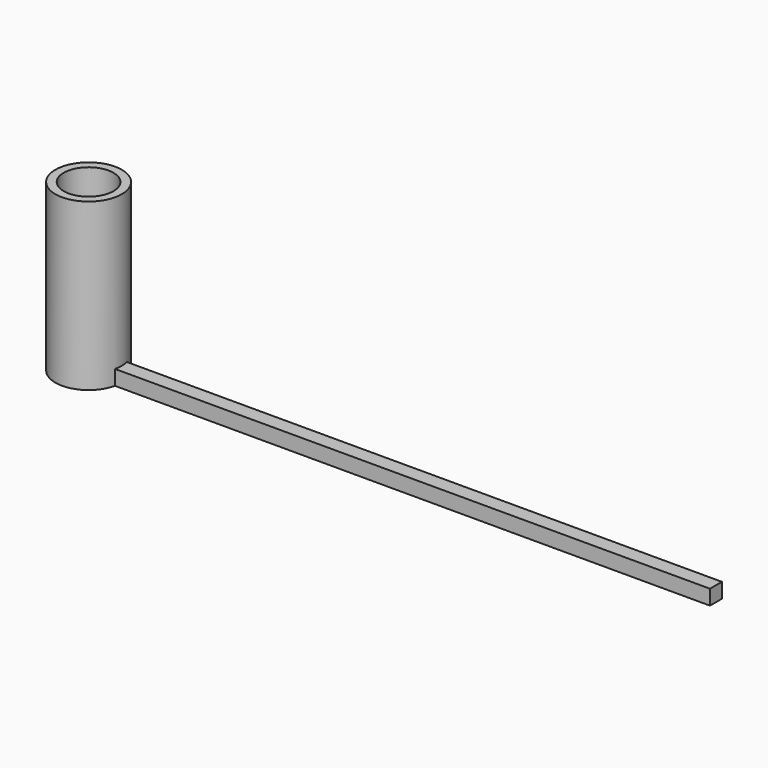
from build123d import *

# Parameters (mm, degrees)
F0_R     = 100
F1_DEPTH = 500
F2_R     = 75
F3_DEPTH = 500.001
F4_W     = 45
F4_H     = 45
F5_DEPTH = 1890
F7_DEPTH = 500.001


with BuildPart() as f1:
    # F0 (on Top) → F1 (new body)
    with BuildSketch(Plane.XY):
        Circle(F0_R)
    extrude(amount=F1_DEPTH)

    # F2 (on face) → F3 (cut, through all)
    with BuildSketch(Plane.XY.offset(500)):
        Circle(F2_R)
    extrude(amount=-F3_DEPTH, mode=Mode.SUBTRACT)

    # F4 (on Right) → F5 (join)
    with BuildSketch(Plane.YZ):
        with Locations((0, 22.5)):
            Rectangle(F4_W, F4_H)
    extrude(amount=F5_DEPTH)

    # F6 (on face) → F7 (cut, through all)
    with BuildSketch(Plane(origin=(0, 0, 0), x_dir=(1, 0, 0), z_dir=(0, 0, -1))):
        with BuildLine():
            ThreePointArc((71.5454401063, -22.5), (74.1313294362, -11.3818274462), (75, 0))
            ThreePointArc((75, 0), (74.1313294362, 11.3818274462), (71.5454401063, 22.5))
            Line((71.5454401063, 22.5), (0, 22.5))
            Line((0, 22.5), (0, -22.5))
            Line((0, -22.5), (71.5454401063, -22.5))
        make_face()
    extrude(amount=-F7_DEPTH, mode=Mode.SUBTRACT)


solid = f1.part
